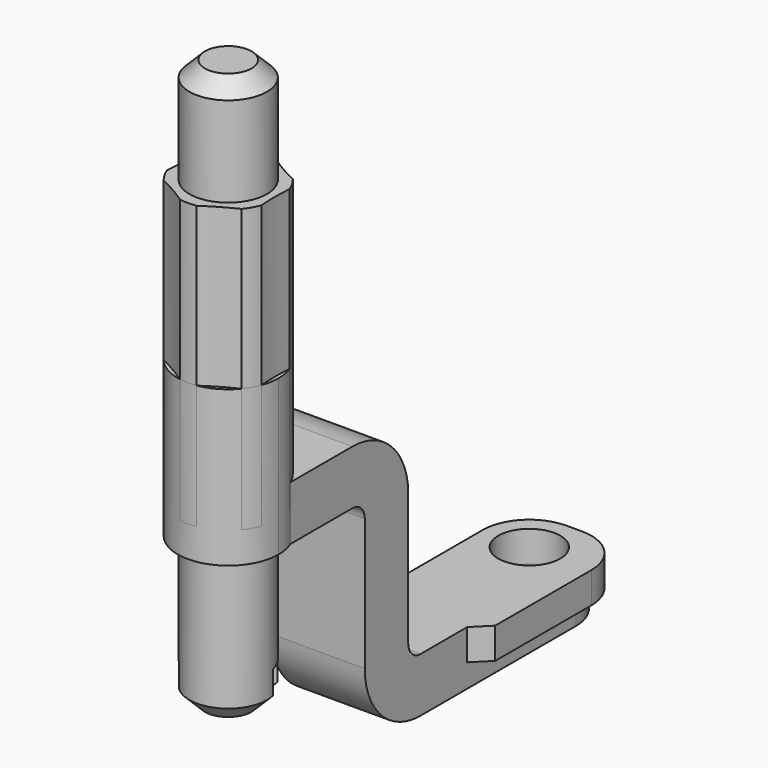
from build123d import *
from build123d import SkipClean  # not in build123d's __all__

# Parameters (mm, degrees)
F0_R      = 2.5
F1_DEPTH  = 36.5
F3_START  = 9.5
F2_R      = 3.25
F3_DEPTH  = 10
F5_DEPTH  = 3
F7_START  = -6.8
F7_DEPTH  = 18.2
F8_R      = 2
F9_DEPTH  = 3.501
F10_R     = 2.99999
F12_DEPTH = 2.5
F13_SIZE  = 0.9999
F14_R     = 2
F15_DEPTH = 2


# Not quite as in the source:
# - a fillet or chamfer is up to 0.001 mm smaller than in the source, because OpenCascade refuses the exact size
# - after a boolean that leaves OpenCascade's solid faulty, fix() repairs it
# - ends of sketch curves that miss each other by under 0.0002 mm in the source are joined


with BuildPart() as f1:
    # F0 (on Top) → F1 (new body)
    with BuildSketch(Plane.XY):
        Circle(F0_R)
    extrude(amount=F1_DEPTH)

    # F2 (on Top) → F3 (join)
    with BuildSketch(Plane.XY.offset(F3_START)):
        Circle(F2_R)
    extrude(amount=F3_DEPTH)

    # F4 (on Right) → F5 (join, symmetric)
    with BuildSketch(Plane.YZ):
        with BuildLine():
            Line((0, 13), (0, 9.5))
            Line((0, 9.5), (6.25, 9.5))
            ThreePointArc((6.25, 9.5), (6.9571067812, 9.2071067812), (7.25, 8.5))
            Line((7.25, 8.5), (7.25, 0))
            ThreePointArc((7.25, 0), (8.5680194847, -3.1819805153), (11.75, -4.5))
            Line((11.75, -4.5), (27.25, -4.5))
            Line((27.25, -4.5), (27.25, -1))
            Line((27.25, -1), (11.75, -1))
            ThreePointArc((11.75, -1), (11.0428932188, -0.7071067812), (10.75, 0))
            Line((10.75, 0), (10.75, 8.5))
            ThreePointArc((10.75, 8.5), (9.4319805153, 11.6819805153), (6.25, 13))
            Line((6.25, 13), (0, 13))
        make_face()
    extrude(amount=F5_DEPTH, both=True)

    # F6 (on face) → F7 (join)
    with BuildSketch(Plane.XY.offset(36.5).offset(F7_START)):
        with BuildLine():
            ThreePointArc((3.0434027778, -1.1402629224), (3, 0), (3.0434027778, 1.1402629224))
            ThreePointArc((3.0434027778, 1.1402629224), (2.8145825623, 1.625), (2.5091980467, 2.0655326583))
            ThreePointArc((2.5091980467, 2.0655326583), (1.5, 2.5980762114), (0.5342047311, 3.2057955807))
            ThreePointArc((0.5342047311, 3.2057955807), (0, 3.25), (-0.5342047311, 3.2057955807))
            ThreePointArc((-0.5342047311, 3.2057955807), (-1.5, 2.5980762114), (-2.5091980467, 2.0655326583))
            ThreePointArc((-2.5091980467, 2.0655326583), (-2.8145825623, 1.625), (-3.0434027778, 1.1402629224))
            ThreePointArc((-3.0434027778, 1.1402629224), (-3, 0), (-3.0434027778, -1.1402629224))
            ThreePointArc((-3.0434027778, -1.1402629224), (-2.8145825623, -1.625), (-2.5091980467, -2.0655326583))
            ThreePointArc((-2.5091980467, -2.0655326583), (-1.5, -2.5980762114), (-0.5342047311, -3.2057955807))
            ThreePointArc((-0.5342047311, -3.2057955807), (0, -3.25), (0.5342047311, -3.2057955807))
            ThreePointArc((0.5342047311, -3.2057955807), (1.5, -2.5980762114), (2.5091980467, -2.0655326583))
            ThreePointArc((2.5091980467, -2.0655326583), (2.8145825623, -1.625), (3.0434027778, -1.1402629224))
        make_face()
    with SkipClean():  # cleaning this boolean's faces spoils the solid; the shape is the same uncleaned
        extrude(amount=-F7_DEPTH)

    # F8 (on face) → F9 (cut, through all)
    with BuildSketch(Plane.XY.offset(-1)):
        with Locations((0, 24.25)):
            Circle(F8_R)
    extrude(amount=-F9_DEPTH, mode=Mode.SUBTRACT)

    add(f1.part.fix(), mode=Mode.REPLACE)

    # F10 (radius 3 in the source; OpenCascade refuses exactly that, so slightly less here)
    f10_edges = [f1.edges().sort_by_distance(p)[0] for p in [
        (-3, 27.25, -2.75),
        (3, 27.25, -2.75),
    ]]
    fillet(f10_edges, radius=F10_R)

    # F11 (on face) → F12 (cut)
    with BuildSketch(Plane(origin=(0, 0, 0), x_dir=(1, 0, 0), z_dir=(0, 0, -1))):
        with BuildLine():
            ThreePointArc((1.6903389552, -1.8419430546), (2.1650635095, -1.25), (2.4403389552, -0.5429049489))
            Line((2.4403389552, -0.5429049489), (-1.6903389552, 1.8419430546))
            ThreePointArc((-1.6903389552, 1.8419430546), (-2.1650635095, 1.25), (-2.4403389552, 0.5429049489))
            Line((-2.4403389552, 0.5429049489), (1.6903389552, -1.8419430546))
        make_face()
    extrude(amount=-F12_DEPTH, mode=Mode.SUBTRACT)

    # F13 (size 1 in the source; OpenCascade refuses exactly that, so slightly less here)
    f13_edges = [f1.edges().sort_by_distance(p)[0] for p in [
        (-1.25, 2.165064, 0),
        (-2.5, 0, 36.5),
        (1.00602, -2.288651, 0),
    ]]
    chamfer(f13_edges, length=F13_SIZE)

    # F14 (on face) → F15 (join)
    with BuildSketch(Plane.XY.offset(-1)):
        with BuildLine():
            Line((3, 24.25), (3, 15.5))
            Line((3, 15.5), (4, 16.5))
            Line((4, 16.5), (4, 24.25))
            ThreePointArc((4, 24.25), (3.1213203436, 26.3713203436), (1, 27.25))
            Line((1, 27.25), (0, 27.25))
            ThreePointArc((0, 27.25), (2.1213203436, 26.3713203436), (3, 24.25))
        make_face()
        with BuildLine():
            Line((3, 11.75), (3, 15.5))
            Line((3, 15.5), (3, 24.25))
            ThreePointArc((3, 24.25), (2.1213203436, 26.3713203436), (0, 27.25))
            ThreePointArc((0, 27.25), (-2.1213232725, 26.3713232725), (-3, 24.25001))
            Line((-3, 24.25001), (-3, 11.75))
            Line((-3, 11.75), (3, 11.75))
        make_face()
        with Locations((0, 24.25)):
            Circle(F14_R, mode=Mode.SUBTRACT)
    extrude(amount=-F15_DEPTH)


solid = f1.part
